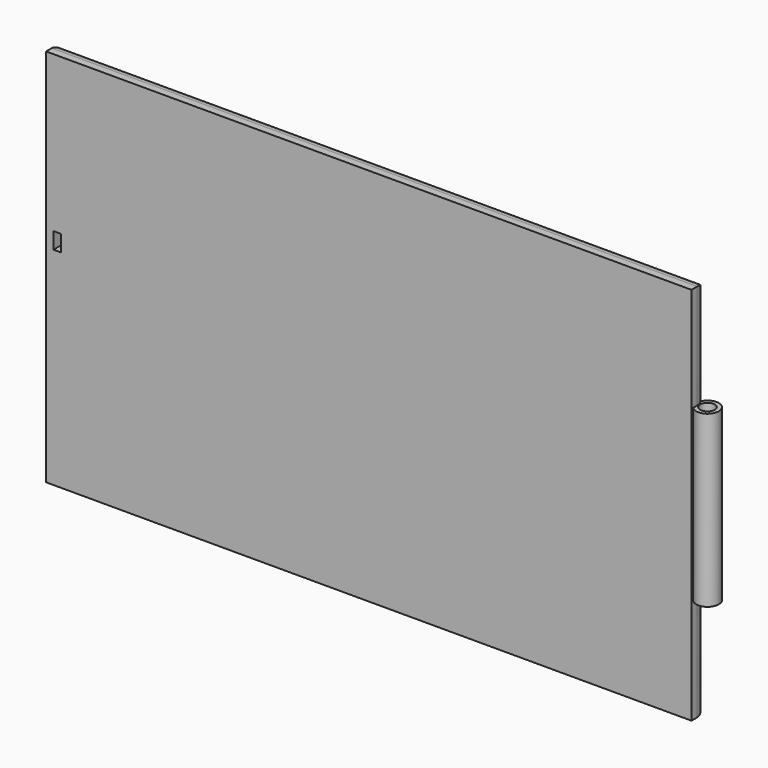
from build123d import *

# Parameters (mm, degrees)
F0_W          = 123.7234
F0_H          = 72.7202
F1_DEPTH      = 3.81
F2_R          = 2.159
F2_R_2        = 1.397
F3_DEPTH      = 72.7202
F4_R          = 1.397
F5_DEPTH      = 20.066
F6_R          = 1.397
F7_DEPTH      = 20.066
F8_W          = 1.4323815703
F8_H          = 3.1365510076
F9_DEPTH      = 25.4
F10_T1_DEPTH  = 135.9876048969
F10_T3_DEPTH  = 84.9844048969
F10_T8_DEPTH  = 84.9844048969
F10_S10_R     = 2.159
F10_T11_DEPTH = 44
F10_T15_DEPTH = 84.9844048969
F10_S17_R     = 2.159
F10_T18_DEPTH = 44
F10_T22_DEPTH = 84.9844048969
F10_S24_R     = 2.159
F10_T25_DEPTH = 44
F10_T30_DEPTH = 84.9844048969
F10_S31_R     = 2.159
F10_T32_DEPTH = 44
F10_T37_DEPTH = 84.9844048969
F10_S38_R     = 2.159
F10_T39_DEPTH = 44


# Not quite as in the source:
# - a fillet or chamfer that OpenCascade refuses, or shapes differently, is made with other operations: its cross-section is extruded or revolved along the edge and cut away or added


with BuildPart() as f1:
    # F0 (on Front) → F1 (new body)
    with BuildSketch(Plane.XZ):
        with Locations((-21.517843008, 12.1004326615)):
            Rectangle(F0_W, F0_H)
    extrude(amount=F1_DEPTH)

    # F2 (on face) → F3 (join)
    with BuildSketch(Plane(origin=(0, 0, -24.2596673385), x_dir=(1, 0, 0), z_dir=(0, 0, -1))):
        with Locations((41.893256992, 1.905)):
            Circle(F2_R)
        with Locations((41.893256992, 1.905)):
            Circle(F2_R_2, mode=Mode.SUBTRACT)
    extrude(amount=-F3_DEPTH)

    # F4 (on face) → F5 (cut)
    with BuildSketch(Plane(origin=(0, 0, -24.2596673385), x_dir=(1, 0, 0), z_dir=(0, 0, -1))):
        with BuildLine():
            ThreePointArc((40.343856992, 0.4014573036), (44.052256992, 1.905), (40.343856992, 3.4085426964))
            Line((40.343856992, 3.4085426964), (40.343856992, 0.4014573036))
        make_face()
        with Locations((41.893256992, 1.905)):
            Circle(F4_R, mode=Mode.SUBTRACT)
    extrude(amount=-F5_DEPTH, mode=Mode.SUBTRACT)

    # F6 (on face) → F7 (cut)
    with BuildSketch(Plane.XY.offset(48.4605326615)):
        with BuildLine():
            ThreePointArc((40.343856992, -3.4085426964), (44.052256992, -1.905), (40.343856992, -0.4014573036))
            Line((40.343856992, -0.4014573036), (40.343856992, -3.4085426964))
        make_face()
        with Locations((41.893256992, -1.905)):
            Circle(F6_R, mode=Mode.SUBTRACT)
    extrude(amount=-F7_DEPTH, mode=Mode.SUBTRACT)

    # F8 (on face) → F9 (cut)
    with BuildSketch(Plane(origin=(0, 0, 0), x_dir=(-1, 0, 0), z_dir=(0, 1, 0))):
        with Locations((81.2400989234, 17.0341590419)):
            Rectangle(F8_W, F8_H)
    extrude(amount=-F9_DEPTH, mode=Mode.SUBTRACT)

    # F10: fillet of radius 2.4528409794 on 4 edges, made by hand

    # F10_s2 → F10_t1 (cut)
    with BuildSketch(Plane.YZ.offset(-89.5116454565)):
        with BuildLine():
            ThreePointArc((-2.4528409794, 48.4605326615), (-0.7184204897, 47.7421121718), (0, 46.0076916821))
            Line((0, 46.0076916821), (0, 48.4605326615))
            Line((0, 48.4605326615), (-2.4528409794, 48.4605326615))
        make_face()
        with BuildLine():
            ThreePointArc((-2.4528409794, -24.2596673385), (-0.7184204897, -23.5412468488), (0, -21.8068263591))
            Line((0, -21.8068263591), (0, -24.2596673385))
            Line((0, -24.2596673385), (-2.4528409794, -24.2596673385))
        make_face()
    extrude(amount=F10_T1_DEPTH, mode=Mode.SUBTRACT)

    # F10_s4 → F10_t3 (cut)
    with BuildSketch(Plane.XY.offset(-30.3917697869)):
        with BuildLine():
            ThreePointArc((-83.379543008, -2.4528409794), (-82.6611225184, -0.7184204897), (-80.9267020287, 0))
            Line((-80.9267020287, 0), (-83.379543008, 0))
            Line((-83.379543008, 0), (-83.379543008, -2.4528409794))
        make_face()
    extrude(amount=F10_T3_DEPTH, mode=Mode.SUBTRACT)


with BuildPart() as f10_tool6:
    # F10_s7 → F10_t8 (new body)
    with BuildSketch(Plane.XY.offset(-30.3917697869)):
        with BuildLine():
            ThreePointArc((37.8910160126, 0), (39.6254365023, -0.7184204897), (40.343856992, -2.4528409794))
            Line((40.343856992, -2.4528409794), (40.343856992, 0))
            Line((40.343856992, 0), (37.8910160126, 0))
        make_face()
    extrude(amount=F10_T8_DEPTH)

    split(bisect_by=Plane.XY.offset(-4.1936673385), keep=Keep.BOTTOM)

    # F10_s10 → F10_t11 (cut, symmetric)
    with BuildSketch(Plane.XY.offset(12.1)):
        with Locations((41.893256992, -1.905)):
            Circle(F10_S10_R)
    extrude(amount=F10_T11_DEPTH, both=True, mode=Mode.SUBTRACT)


with BuildPart() as f1_1:
    add(f1.part)

    # F10_t5: cut F10_tool6
    add(f10_tool6.part, mode=Mode.SUBTRACT)


with BuildPart() as f10_tool13:
    # F10_s14 → F10_t15 (new body)
    with BuildSketch(Plane.XY.offset(-30.3917697869)):
        with BuildLine():
            ThreePointArc((37.8910160126, 0), (39.6254365023, -0.7184204897), (40.343856992, -2.4528409794))
            Line((40.343856992, -2.4528409794), (40.343856992, 0))
            Line((40.343856992, 0), (37.8910160126, 0))
        make_face()
    extrude(amount=F10_T15_DEPTH)

    split(bisect_by=Plane.XY.offset(-4.1936673385), keep=Keep.BOTTOM)

    # F10_s17 → F10_t18 (intersect, symmetric)
    with BuildSketch(Plane.XY.offset(12.1)):
        with Locations((41.893256992, -1.905)):
            Circle(F10_S17_R)
    extrude(amount=F10_T18_DEPTH, both=True, mode=Mode.INTERSECT)


with BuildPart() as f1_2:
    add(f1_1.part)

    # F10_t12: cut F10_tool13
    add(f10_tool13.part, mode=Mode.SUBTRACT)


with BuildPart() as f10_tool20:
    # F10_s21 → F10_t22 (new body)
    with BuildSketch(Plane.XY.offset(-30.3917697869)):
        with BuildLine():
            ThreePointArc((37.8910160126, 0), (39.6254365023, -0.7184204897), (40.343856992, -2.4528409794))
            Line((40.343856992, -2.4528409794), (40.343856992, 0))
            Line((40.343856992, 0), (37.8910160126, 0))
        make_face()
    extrude(amount=F10_T22_DEPTH)

    split(bisect_by=Plane.XY.offset(-4.1936673385), keep=Keep.TOP)

    # F10_s24 → F10_t25 (cut, symmetric)
    with BuildSketch(Plane.XY.offset(12.1)):
        with Locations((41.893256992, -1.905)):
            Circle(F10_S24_R)
    extrude(amount=F10_T25_DEPTH, both=True, mode=Mode.SUBTRACT)

    split(bisect_by=Plane.XY.offset(28.3945326615), keep=Keep.BOTTOM)


with BuildPart() as f1_3:
    add(f1_2.part)

    # F10_t19: cut F10_tool20
    add(f10_tool20.part, mode=Mode.SUBTRACT)


with BuildPart() as f10_tool28:
    # F10_s29 → F10_t30 (new body)
    with BuildSketch(Plane.XY.offset(-30.3917697869)):
        with BuildLine():
            ThreePointArc((37.8910160126, 0), (39.6254365023, -0.7184204897), (40.343856992, -2.4528409794))
            Line((40.343856992, -2.4528409794), (40.343856992, 0))
            Line((40.343856992, 0), (37.8910160126, 0))
        make_face()
    extrude(amount=F10_T30_DEPTH)

    # F10_s31 → F10_t32 (cut, symmetric)
    with BuildSketch(Plane.XY.offset(12.1)):
        with Locations((41.893256992, -1.905)):
            Circle(F10_S31_R)
    extrude(amount=F10_T32_DEPTH, both=True, mode=Mode.SUBTRACT)

    split(bisect_by=Plane.XY.offset(28.3945326615), keep=Keep.TOP)


with BuildPart() as f1_4:
    add(f1_3.part)

    # F10_t27: cut F10_tool28
    add(f10_tool28.part, mode=Mode.SUBTRACT)


with BuildPart() as f10_tool35:
    # F10_s36 → F10_t37 (new body)
    with BuildSketch(Plane.XY.offset(-30.3917697869)):
        with BuildLine():
            ThreePointArc((37.8910160126, 0), (39.6254365023, -0.7184204897), (40.343856992, -2.4528409794))
            Line((40.343856992, -2.4528409794), (40.343856992, 0))
            Line((40.343856992, 0), (37.8910160126, 0))
        make_face()
    extrude(amount=F10_T37_DEPTH)

    # F10_s38 → F10_t39 (intersect, symmetric)
    with BuildSketch(Plane.XY.offset(12.1)):
        with Locations((41.893256992, -1.905)):
            Circle(F10_S38_R)
    extrude(amount=F10_T39_DEPTH, both=True, mode=Mode.INTERSECT)

    split(bisect_by=Plane.XY.offset(28.3945326615), keep=Keep.TOP)


with BuildPart() as f1_5:
    add(f1_4.part)

    # F10_t34: cut F10_tool35
    add(f10_tool35.part, mode=Mode.SUBTRACT)


solid = f1_5.part
